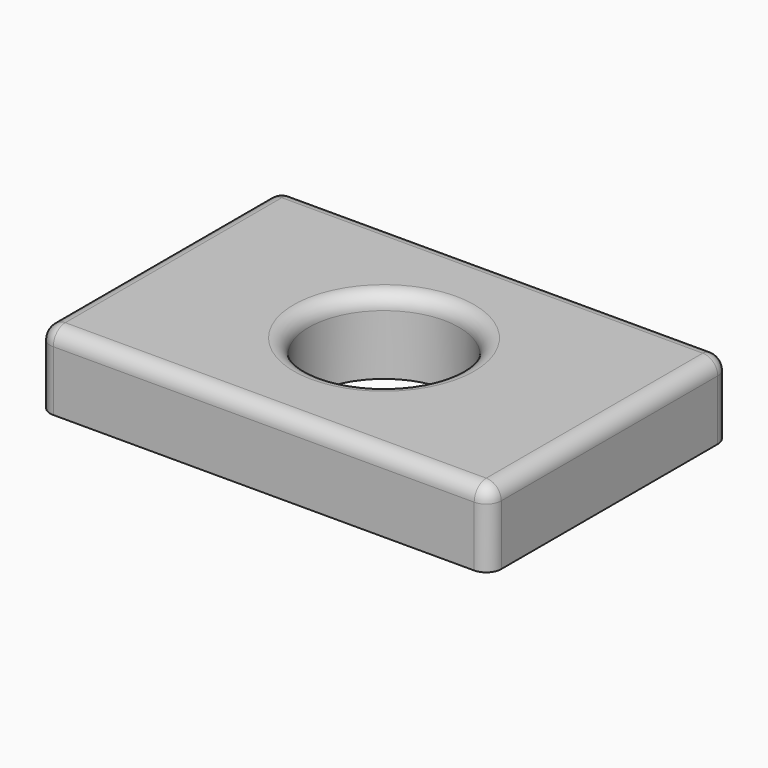
from build123d import *

# Parameters (mm, degrees)
F0_W     = 76.2
F0_H     = 50.8
F0_R     = 12.7
F1_DEPTH = 12.7
F2_R     = 2.54
F3_T     = 2.54


# Not quite as in the source:
# - a shell that OpenCascade refuses in one call is made with other operations: the cavity is built on its own and cut out


with BuildPart() as f1:
    # F0 (on Top) → F1 (new body)
    with BuildSketch(Plane.XY):
        Rectangle(F0_W, F0_H)
        Circle(F0_R, mode=Mode.SUBTRACT)
    extrude(amount=F1_DEPTH)

    # F2
    f2_edges = [f1.edges().sort_by_distance(p)[0] for p in [
        (-38.1, -25.4, 6.35),
        (38.1, -25.4, 6.35),
        (38.1, 25.4, 6.35),
        (-38.1, 25.4, 6.35),
        (0, 25.4, 12.7),
        (-38.1, 0, 12.7),
        (0, -25.4, 12.7),
        (38.1, 0, 12.7),
        (-12.7, 0, 12.7),
    ]]
    fillet(f2_edges, radius=F2_R)

    # F3: shell of thickness 2.54, made by hand


with BuildPart() as f3_core1:
    # F3_t2: copy of F1
    add(f1.part)

    # the walls: a layer under each face that stays
    f3_faces = [f3_core1.faces().sort_by_distance(p)[0] for p in [
        (38.1, 0, 5.08),
        (0, -25.4, 5.08),
        (0, 25.4, 5.08),
        (-38.1, 0, 5.08),
        (-12.7, 0, 5.08),
        (-23.7066666667, -15.24, 12.7),
    ]]
    thicken(f3_faces, amount=-F3_T, mode=Mode.SUBTRACT)


with BuildPart() as f1_1:
    add(f1.part)

    # what is left inside the walls is the cavity
    f3_cavity = [f3_core1.part.solids().sort_by_distance(p)[0] for p in [
        (-17.78, 7.62, 0.0254),
    ]]
    add(f3_cavity, mode=Mode.SUBTRACT)


solid = f1_1.part
